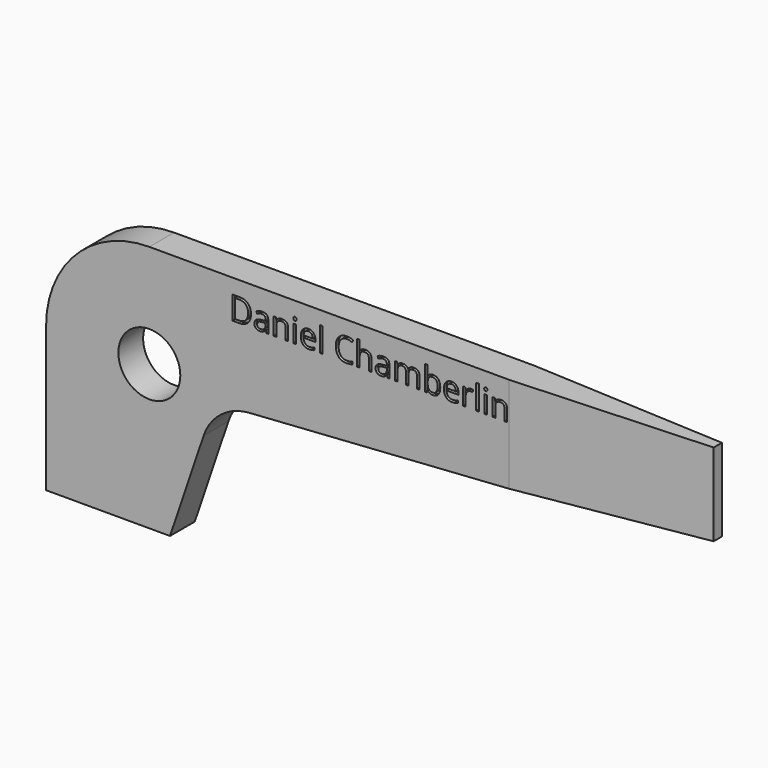
from build123d import *

# Parameters (mm, degrees)
F1_DEPTH     = 2.38125
F2_R         = 2.38125
F3_DEPTH     = 25.4
F4_DEPTH     = 25.4
F5_R         = 2.38125
F6_DEPTH     = 25.4
F8_DEPTH     = 25.4
F9_TEXT_SIZE = 2.489583277
F10_DEPTH    = 0.254


# Not quite as in the source:
# - Text() gives the source's letters only with a copy of the font that has no kerning and outlines rounded to 1/6400 em; it was checked with that copy


with BuildPart() as f1:
    # F0 (on Front) → F1 (new body)
    with BuildSketch(Plane.XZ):
        with BuildLine():
            Line((50.6850704551, 19.05), (7.9375, 19.05))
            ThreePointArc((7.9375, 19.05), (2.3248399243, 16.7251600757), (0, 11.1125))
            Line((0, 11.1125), (0, 0))
            Line((0, 0), (9.525, 0))
            Line((9.525, 0), (12.1103451907, 7.6262422093))
            ThreePointArc((12.1103451907, 7.6262422093), (13.4506862777, 9.5002576063), (15.6054695585, 10.3159517585))
            Line((15.6054695585, 10.3159517585), (50.6850704551, 12.7))
            Line((50.6850704551, 12.7), (50.6850704551, 19.05))
        make_face()
    extrude(amount=F1_DEPTH)

    # F2 (on face) → F3 (join)
    with BuildSketch(Plane.XZ.offset(2.38125)):
        with Locations((7.9502, 11.1125)):
            Circle(F2_R)
    extrude(amount=F3_DEPTH)

    # F4 (cut): a face of the model
    f4_faces = [f1.faces().sort_by_distance(p)[0] for p in [
        (7.9502, -27.78125, 11.1125),
    ]]
    extrude(f4_faces, amount=-F4_DEPTH, mode=Mode.SUBTRACT)

    # F5 (on face) → F6 (cut)
    with BuildSketch(Plane.XZ.offset(2.38125)):
        with Locations((7.9375, 11.1125)):
            Circle(F5_R)
    extrude(amount=-F6_DEPTH, mode=Mode.SUBTRACT)

    # F7 (on face) → F8 (cut)
    with BuildSketch(Plane.XY.offset(19.05)):
        Polygon((50.6850704551, 0), (35.6038204551, 0), (50.6850704551, -0.79375), align=None)
        Polygon((50.6850704551, -2.38125), (50.6850704551, -1.5875), (35.6038204551, -2.38125), align=None)
    extrude(amount=-F8_DEPTH, mode=Mode.SUBTRACT)

    # F9 (on face) → F10 (cut)
    with BuildSketch(Plane.XZ.offset(2.38125)):
        with Locations((14.0864299917, 16.1319189114)):
            Text('Daniel Chamberlin', F9_TEXT_SIZE, font='Open Sans', text_align=(TextAlign.LEFT, TextAlign.BOTTOM))
    extrude(amount=-F10_DEPTH, mode=Mode.SUBTRACT)


solid = f1.part
